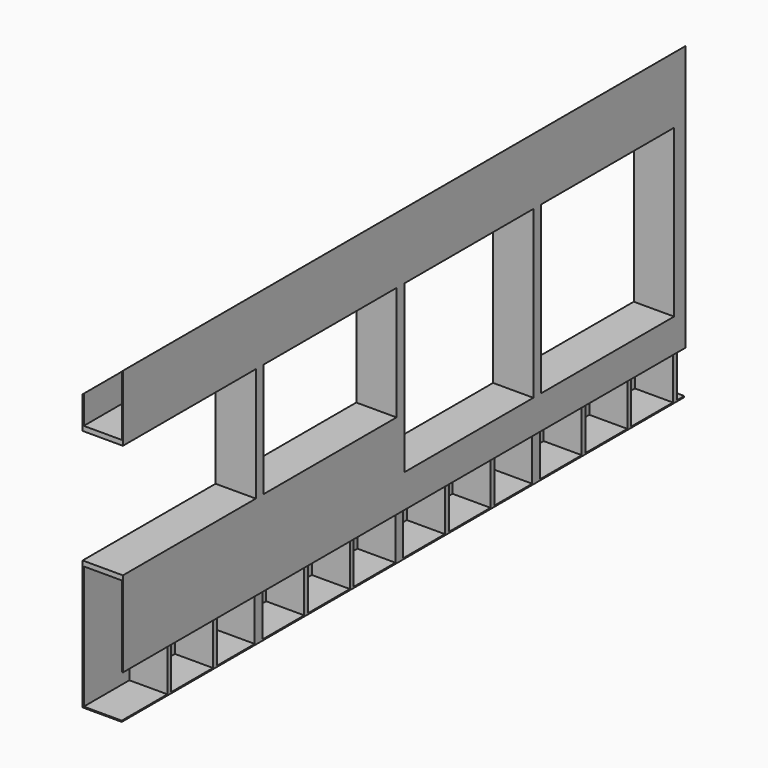
from build123d import *

# Parameters (mm, degrees)
F0_W     = 51
F0_H     = 749
F0_H_2   = 1299
F0_H_3   = 699
F1_DEPTH = 400
F2_W     = 98
F2_H     = 3200
F2_W_2   = 549
F2_H_2   = 749
F2_W_3   = 498
F2_H_3   = 1299
F2_W_4   = 600
F2_H_4   = 599
F2_W_5   = 1749
F2_H_5   = 1750
F2_W_6   = 1698
F2_H_6   = 1200
F3_DEPTH = 12
F4_W     = 549
F4_H     = 699
F4_W_2   = 498
F4_W_3   = 600
F4_W_4   = 98
F4_H_2   = 2850
F4_H_3   = 849
F4_H_4   = 299
F4_W_5   = 1749
F4_H_5   = 1200
F4_W_6   = 1698
F4_H_6   = 1750
F5_DEPTH = 12
F6_W     = 400
F6_H     = 7400
F7_DEPTH = 12
F9_DEPTH = 7400.001


# Not quite as in the source:
# - a feature names something its author has since deleted; it is built from what else it names


with BuildPart() as f1:
    # F0 (on Right) → F1 (new body)
    with BuildSketch(Plane.YZ):
        Polygon((-149, 0), (-98, 0), (-98, 3300), (-149, 3300), (-149, 2601), (-149, 2550), (-149, 800), (-149, 749), align=None)
        with Locations((-1323.5, 374.5)):
            Rectangle(F0_W, F0_H)
        with Locations((-2523.5, 374.5)):
            Rectangle(F0_W, F0_H)
        with Locations((-3123.5, 374.5)):
            Rectangle(F0_W, F0_H)
        with Locations((-4374.5, 649.5)):
            Rectangle(F0_W, F0_H_2)
        with Locations((-4974.5, 649.5)):
            Rectangle(F0_W, F0_H_2)
        with Locations((-6174.5, 649.5)):
            Rectangle(F0_W, F0_H_2)
        with Locations((-6774.5, 649.5)):
            Rectangle(F0_W, F0_H_2)
        with Locations((-1323.5, 2950.5)):
            Rectangle(F0_W, F0_H_3)
        with Locations((-2523.5, 2950.5)):
            Rectangle(F0_W, F0_H_3)
        with Locations((-3123.5, 2950.5)):
            Rectangle(F0_W, F0_H_3)
        with Locations((-4374.5, 2950.5)):
            Rectangle(F0_W, F0_H_3)
        with Locations((-4974.5, 2950.5)):
            Rectangle(F0_W, F0_H_3)
        with Locations((-6174.5, 2950.5)):
            Rectangle(F0_W, F0_H_3)
        with Locations((-6774.5, 2950.5)):
            Rectangle(F0_W, F0_H_3)
        with Locations((-723.5, 374.5)):
            Rectangle(F0_W, F0_H)
        Polygon((-1898, 749), (-1898, 800), (-1898, 2550), (-1898, 2601), (-1898, 3300), (-1949, 3300), (-1949, 0), (-1898, 0), align=None)
        Polygon((-2000, 0), (-1949, 0), (-1949, 3300), (-2000, 3300), (-2000, 2601), (-2000, 2550), (-2000, 800), (-2000, 749), align=None)
        Polygon((-3698, 749), (-3698, 800), (-3698, 2550), (-3698, 2601), (-3698, 3300), (-3749, 3300), (-3749, 0), (-3698, 0), align=None)
        Polygon((-3800, 0), (-3749, 0), (-3749, 3300), (-3800, 3300), (-3800, 2601), (-3800, 2550), (-3800, 1350), (-3800, 1299), align=None)
        Polygon((-5549, 1299), (-5549, 1350), (-5549, 2550), (-5549, 2601), (-5549, 3300), (-5600, 3300), (-5600, 0), (-5549, 0), align=None)
        Polygon((-5651, 0), (-5600, 0), (-5600, 3300), (-5651, 3300), (-5651, 2601), (-5651, 2550), (-5651, 1350), (-5651, 1299), align=None)
        Polygon((-6149, 1299), (-5651, 1299), (-5651, 1350), (-7400, 1350), (-7400, 1299), (-6800, 1299), (-6749, 1299), (-6200, 1299), align=None)
        Polygon((-5651, 2550), (-5651, 2601), (-6149, 2601), (-6200, 2601), (-6749, 2601), (-6800, 2601), (-7400, 2601), (-7400, 2550), align=None)
        Polygon((-698, 749), (-149, 749), (-149, 800), (-1898, 800), (-1898, 749), (-1349, 749), (-1298, 749), (-749, 749), align=None)
        Polygon((-2498, 749), (-2000, 749), (-2000, 800), (-3698, 800), (-3698, 749), (-3149, 749), (-3098, 749), (-2549, 749), align=None)
        Polygon((-4349, 1299), (-3800, 1299), (-3800, 1350), (-5549, 1350), (-5549, 1299), (-5000, 1299), (-4949, 1299), (-4400, 1299), align=None)
        Polygon((-3800, 2550), (-3800, 2601), (-4349, 2601), (-4400, 2601), (-4949, 2601), (-5000, 2601), (-5549, 2601), (-5549, 2550), align=None)
        Polygon((-149, 2550), (-149, 2601), (-698, 2601), (-749, 2601), (-1298, 2601), (-1349, 2601), (-1898, 2601), (-1898, 2550), align=None)
        Polygon((-2000, 2550), (-2000, 2601), (-2498, 2601), (-2549, 2601), (-3098, 2601), (-3149, 2601), (-3698, 2601), (-3698, 2550), align=None)
        with Locations((-723.5, 2950.5)):
            Rectangle(F0_W, F0_H_3)
    extrude(amount=F1_DEPTH)

    # F2 (on face) → F3 (join)
    with BuildSketch(Plane(origin=(0, 0, 0), x_dir=(0, -1, 0), z_dir=(-1, 0, 0))):
        with Locations((49, 1600)):
            Rectangle(F2_W, F2_H)
        with Locations((1023.5, 374.5)):
            Rectangle(F2_W_2, F2_H_2)
        with Locations((1623.5, 374.5)):
            Rectangle(F2_W_2, F2_H_2)
        with Locations((2249, 374.5)):
            Rectangle(F2_W_3, F2_H_2)
        with Locations((2823.5, 374.5)):
            Rectangle(F2_W_2, F2_H_2)
        with Locations((3423.5, 374.5)):
            Rectangle(F2_W_2, F2_H_2)
        with Locations((4074.5, 649.5)):
            Rectangle(F2_W_2, F2_H_3)
        with Locations((4674.5, 649.5)):
            Rectangle(F2_W_2, F2_H_3)
        with Locations((5274.5, 649.5)):
            Rectangle(F2_W_2, F2_H_3)
        with Locations((5900, 649.5)):
            Rectangle(F2_W_3, F2_H_3)
        with Locations((6474.5, 649.5)):
            Rectangle(F2_W_2, F2_H_3)
        with Locations((7100, 649.5)):
            Rectangle(F2_W_4, F2_H_3)
        with Locations((1023.5, 2900.5)):
            Rectangle(F2_W_2, F2_H_4)
        with Locations((1623.5, 2900.5)):
            Rectangle(F2_W_2, F2_H_4)
        with Locations((2249, 2900.5)):
            Rectangle(F2_W_3, F2_H_4)
        with Locations((2823.5, 2900.5)):
            Rectangle(F2_W_2, F2_H_4)
        with Locations((3423.5, 2900.5)):
            Rectangle(F2_W_2, F2_H_4)
        with Locations((4074.5, 2900.5)):
            Rectangle(F2_W_2, F2_H_4)
        with Locations((4674.5, 2900.5)):
            Rectangle(F2_W_2, F2_H_4)
        with Locations((5274.5, 2900.5)):
            Rectangle(F2_W_2, F2_H_4)
        with Locations((5900, 2900.5)):
            Rectangle(F2_W_3, F2_H_4)
        with Locations((6474.5, 2900.5)):
            Rectangle(F2_W_2, F2_H_4)
        with Locations((7100, 2900.5)):
            Rectangle(F2_W_4, F2_H_4)
        with Locations((423.5, 2900.5)):
            Rectangle(F2_W_2, F2_H_4)
        with Locations((423.5, 374.5)):
            Rectangle(F2_W_2, F2_H_2)
        Polygon((98, 3200), (98, 0), (149, 0), (149, 749), (698, 749), (698, 0), (749, 0), (749, 749), (1298, 749), (1298, 0), (1349, 0), (1349, 749), (1898, 749), (1898, 0), (2000, 0), (2000, 749), (2498, 749), (2498, 0), (2549, 0), (2549, 749), (3098, 749), (3098, 0), (3149, 0), (3149, 749), (3698, 749), (3698, 0), (3800, 0), (3800, 1299), (4349, 1299), (4349, 0), (4400, 0), (4400, 1299), (4949, 1299), (4949, 0), (5000, 0), (5000, 1299), (5549, 1299), (5549, 0), (5651, 0), (5651, 1299), (6149, 1299), (6149, 0), (6200, 0), (6200, 1299), (6749, 1299), (6749, 0), (6800, 0), (6800, 1299), (7400, 1299), (7400, 1350), (5651, 1350), (5651, 2550), (7400, 2550), (7400, 2601), (6800, 2601), (6800, 3200), (6749, 3200), (6749, 2601), (6200, 2601), (6200, 3200), (6149, 3200), (6149, 2601), (5651, 2601), (5651, 3200), (5549, 3200), (5549, 2601), (5000, 2601), (5000, 3200), (4949, 3200), (4949, 2601), (4400, 2601), (4400, 3200), (4349, 3200), (4349, 2601), (3800, 2601), (3800, 3200), (3698, 3200), (3698, 2601), (3149, 2601), (3149, 3200), (3098, 3200), (3098, 2601), (2549, 2601), (2549, 3200), (2498, 3200), (2498, 2601), (2000, 2601), (2000, 3200), (1898, 3200), (1898, 2601), (1349, 2601), (1349, 3200), (1298, 3200), (1298, 2601), (749, 2601), (749, 3200), (698, 3200), (698, 2601), (149, 2601), (149, 3200), align=None)
        with Locations((1023.5, 1675)):
            Rectangle(F2_W_5, F2_H_5, mode=Mode.SUBTRACT)
        with Locations((2849, 1675)):
            Rectangle(F2_W_6, F2_H_5, mode=Mode.SUBTRACT)
        with Locations((4674.5, 1950)):
            Rectangle(F2_W_5, F2_H_6, mode=Mode.SUBTRACT)
    extrude(amount=F3_DEPTH)

    # F4 (on face) → F5 (join)
    with BuildSketch(Plane.YZ.offset(400)):
        with Locations((-1023.5, 2950.5)):
            Rectangle(F4_W, F4_H)
        with Locations((-1623.5, 2950.5)):
            Rectangle(F4_W, F4_H)
        with Locations((-2249, 2950.5)):
            Rectangle(F4_W_2, F4_H)
        with Locations((-2823.5, 2950.5)):
            Rectangle(F4_W, F4_H)
        with Locations((-3423.5, 2950.5)):
            Rectangle(F4_W, F4_H)
        with Locations((-4074.5, 2950.5)):
            Rectangle(F4_W, F4_H)
        with Locations((-4674.5, 2950.5)):
            Rectangle(F4_W, F4_H)
        with Locations((-5274.5, 2950.5)):
            Rectangle(F4_W, F4_H)
        with Locations((-5900, 2950.5)):
            Rectangle(F4_W_2, F4_H)
        with Locations((-6474.5, 2950.5)):
            Rectangle(F4_W, F4_H)
        with Locations((-7100, 2950.5)):
            Rectangle(F4_W_3, F4_H)
        with Locations((-49, 1875)):
            Rectangle(F4_W_4, F4_H_2)
        with Locations((-7100, 874.5)):
            Rectangle(F4_W_3, F4_H_3)
        with Locations((-2249, 599.5)):
            Rectangle(F4_W_2, F4_H_4)
        with Locations((-2823.5, 599.5)):
            Rectangle(F4_W, F4_H_4)
        with Locations((-3423.5, 599.5)):
            Rectangle(F4_W, F4_H_4)
        with Locations((-4074.5, 874.5)):
            Rectangle(F4_W, F4_H_3)
        with Locations((-4674.5, 874.5)):
            Rectangle(F4_W, F4_H_3)
        with Locations((-5274.5, 874.5)):
            Rectangle(F4_W, F4_H_3)
        with Locations((-5900, 874.5)):
            Rectangle(F4_W_2, F4_H_3)
        with Locations((-6474.5, 874.5)):
            Rectangle(F4_W, F4_H_3)
        Polygon((-149, 450), (-98, 450), (-98, 3300), (-149, 3300), (-149, 2601), (-698, 2601), (-698, 3300), (-749, 3300), (-749, 2601), (-1298, 2601), (-1298, 3300), (-1349, 3300), (-1349, 2601), (-1898, 2601), (-1898, 3300), (-2000, 3300), (-2000, 2601), (-2498, 2601), (-2498, 3300), (-2549, 3300), (-2549, 2601), (-3098, 2601), (-3098, 3300), (-3149, 3300), (-3149, 2601), (-3698, 2601), (-3698, 3300), (-3800, 3300), (-3800, 2601), (-4349, 2601), (-4349, 3300), (-4400, 3300), (-4400, 2601), (-4949, 2601), (-4949, 3300), (-5000, 3300), (-5000, 2601), (-5549, 2601), (-5549, 3300), (-5651, 3300), (-5651, 2601), (-6149, 2601), (-6149, 3300), (-6200, 3300), (-6200, 2601), (-6749, 2601), (-6749, 3300), (-6800, 3300), (-6800, 2601), (-7400, 2601), (-7400, 2550), (-5651, 2550), (-5651, 1350), (-7400, 1350), (-7400, 1299), (-6800, 1299), (-6800, 450), (-6749, 450), (-6749, 1299), (-6200, 1299), (-6200, 450), (-6149, 450), (-6149, 1299), (-5651, 1299), (-5651, 450), (-5549, 450), (-5549, 1299), (-5000, 1299), (-5000, 450), (-4949, 450), (-4949, 1299), (-4400, 1299), (-4400, 450), (-4349, 450), (-4349, 1299), (-3800, 1299), (-3800, 450), (-3698, 450), (-3698, 749), (-3149, 749), (-3149, 450), (-3098, 450), (-3098, 749), (-2549, 749), (-2549, 450), (-2498, 450), (-2498, 749), (-2000, 749), (-2000, 450), (-1898, 450), (-1898, 749), (-1349, 749), (-1349, 450), (-1298, 450), (-1298, 749), (-749, 749), (-749, 450), (-698, 450), (-698, 749), (-149, 749), align=None)
        with Locations((-4674.5, 1950)):
            Rectangle(F4_W_5, F4_H_5, mode=Mode.SUBTRACT)
        with Locations((-2849, 1675)):
            Rectangle(F4_W_6, F4_H_6, mode=Mode.SUBTRACT)
        with Locations((-1023.5, 1675)):
            Rectangle(F4_W_5, F4_H_6, mode=Mode.SUBTRACT)
        with Locations((-1623.5, 599.5)):
            Rectangle(F4_W, F4_H_4)
        with Locations((-1023.5, 599.5)):
            Rectangle(F4_W, F4_H_4)
        with Locations((-423.5, 599.5)):
            Rectangle(F4_W, F4_H_4)
        with Locations((-423.5, 2950.5)):
            Rectangle(F4_W, F4_H)
    extrude(amount=F5_DEPTH)

    # F6 (on face) → F7 (join)
    with BuildSketch(Plane(origin=(0, 0, 0), x_dir=(1, 0, 0), z_dir=(0, 0, -1))):
        with Locations((200, 3700)):
            Rectangle(F6_W, F6_H)
        Polygon((-12, 0), (0, 0), (0, 98), (0, 149), (0, 698), (0, 749), (0, 1298), (0, 1349), (0, 1898), (0, 2000), (0, 2498), (0, 2549), (0, 3098), (0, 3149), (0, 3698), (0, 3800), (0, 4349), (0, 4400), (0, 4949), (0, 5000), (0, 5549), (0, 5651), (0, 6149), (0, 6200), (0, 6749), (0, 6800), (0, 7400), (-12, 7400), align=None)
    extrude(amount=F7_DEPTH)

    # F8 (on face) → F9 (cut, through all)
    with BuildSketch(Plane(origin=(0, 0, 0), x_dir=(-1, 0, 0), z_dir=(0, 1, 0))):
        Polygon((-450, 3277.5948340298), (0, 2900), (50, 2858.0450184411), (50, 3377.5948340298), (-450, 3377.5948340298), align=None)
    extrude(amount=-F9_DEPTH, mode=Mode.SUBTRACT)


solid = f1.part
